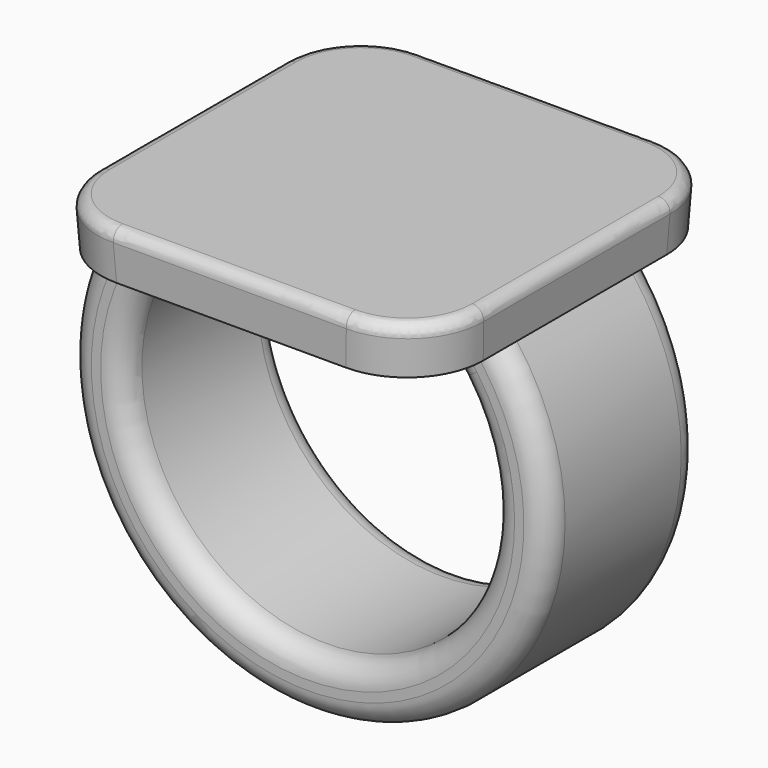
from build123d import *

# Parameters (mm, degrees)
F0_W          = 25.4
F0_H          = 25.4
F1_DEPTH      = 3.175
F1_TAPER      = -3
F3_W          = 5.08
F3_H          = 12.7
F6_DEPTH      = 6.35
F6_DEPTH_BACK = 6.35
F7_R          = 5.08
F8_R          = 1.524
F9_R          = 0.762


with BuildPart() as f1:
    # F0 (on Top) → F1 (new body)
    with BuildSketch(Plane.XY):
        Rectangle(F0_W, F0_H)
    extrude(amount=F1_DEPTH, taper=F1_TAPER)

    # F4: sweep along a path in F2
    with BuildLine(Plane.XZ) as f4_path:
        ThreePointArc((-10.16, 0), (0, -23.5582897328), (10.16, 0))
    # F3 (on face) → F4 (sweep)
    with BuildSketch(Plane(origin=(0, 0, 0), x_dir=(1, 0, 0), z_dir=(0, 0, -1))):
        with Locations((-10.16, 0)):
            Rectangle(F3_W, F3_H)
    sweep(path=f4_path.line)

    # F5 (on Front) → F6 (join, two sides)
    with BuildSketch(Plane.XZ) as f6_sk:
        with BuildLine():
            Line((10.16, 0), (7.62, 0))
            ThreePointArc((7.62, 0), (8.9072265211, -1.1822790439), (10.0130578512, -2.535746045))
            Line((10.0130578512, -2.535746045), (10.16, 0))
        make_face()
    extrude(amount=F6_DEPTH)
    extrude(f6_sk.sketch, amount=-F6_DEPTH_BACK)

    # F7
    f7_edges = [f1.edges().sort_by_distance(p)[0] for p in [
        (-12.783197, 12.783197, 1.5875),
        (-12.783197, -12.783197, 1.5875),
        (12.783197, 12.783197, 1.5875),
        (12.783197, -12.783197, 1.5875),
    ]]
    fillet(f7_edges, radius=F7_R)

    # F8
    f8_edges = [f1.edges().sort_by_distance(p)[0] for p in [
        (-1.743325, -6.35, -21.711017),
        (-1.743325, 6.35, -21.711017),
        (8.907227, 6.35, -1.182279),
        (0, 6.35, -25.501344),
        (8.907227, -6.35, -1.182279),
        (0, -6.35, -25.501344),
    ]]
    fillet(f8_edges, radius=F8_R)

    # F9
    f9_edges = [f1.edges().sort_by_distance(p)[0] for p in [
        (0, 12.866395, 3.175),
        (11.381378, 11.381378, 3.175),
        (-11.381378, 11.381378, 3.175),
        (12.866395, 0, 3.175),
        (-12.866395, 0, 3.175),
        (11.381378, -11.381378, 3.175),
        (-11.381378, -11.381378, 3.175),
        (0, -12.866395, 3.175),
    ]]
    fillet(f9_edges, radius=F9_R)


solid = f1.part
